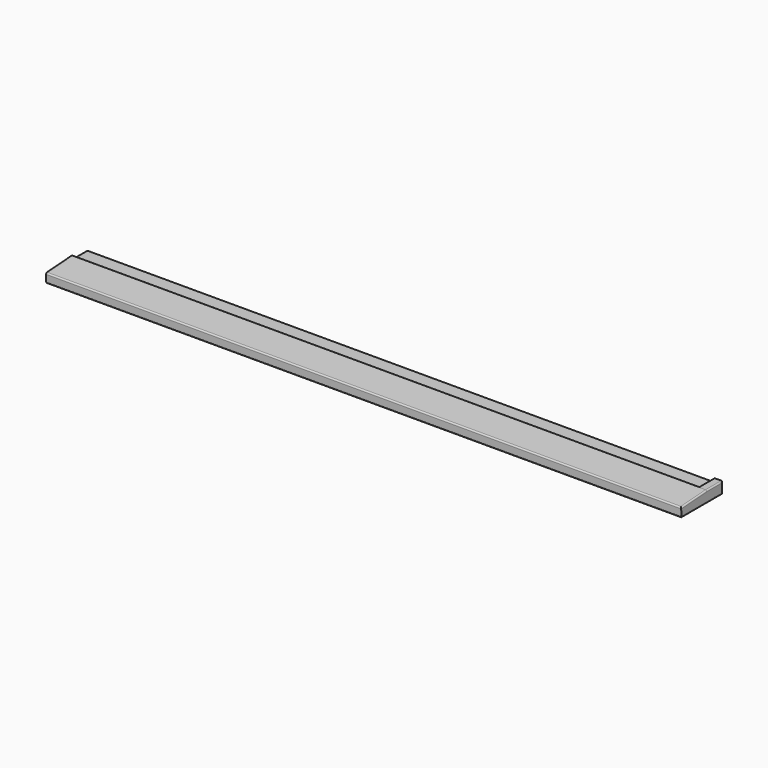
from build123d import *

# Parameters (mm, degrees)
F1_DEPTH    = 2390
F3_DEPTH    = 20
F5_DEPTH    = 10
F6_T1_DEPTH = 216.618628623
F6_T3_DEPTH = 142.4030805268
F6_T5_DEPTH = 100.344113211
F6_T7_DEPTH = 68.9770272469


# Not quite as in the source:
# - a fillet or chamfer that OpenCascade refuses, or shapes differently, is made with other operations: its cross-section is extruded or revolved along the edge and cut away or added


with BuildPart() as f1:
    # F0 (on Right) → F1 (new body)
    with BuildSketch(Plane.YZ):
        with BuildLine():
            Line((0, -19.8239199817), (0, 0))
            Line((0, 0), (190, 0))
            Line((190, 0), (190, 10))
            Line((190, 10), (120, 10))
            Line((120, 10), (120, 19.1649627105))
            ThreePointArc((120, 19.1649627105), (118.4117029432, 22.8201348033), (114.655886789, 24.1531072651))
            Line((114.655886789, 24.1531072651), (-2.4688205766, 16.0731170599))
            ThreePointArc((-2.4688205766, 16.0731170599), (-5.8715951564, 14.3956872139), (-7.1172645938, 10.8122596114))
            Line((-7.1172645938, 10.8122596114), (-6.3410848379, -15.7684031874))
            ThreePointArc((-6.3410848379, -15.7684031874), (-4.7310556973, -18.6708970152), (-1.618628623, -19.8239199817))
            Line((-1.618628623, -19.8239199817), (0, -19.8239199817))
        make_face()
    extrude(amount=-F1_DEPTH)

    # F2 (on face) → F3 (join)
    with BuildSketch(Plane.YZ):
        with BuildLine():
            ThreePointArc((-6.3410848379, -15.7684031874), (-4.7310556973, -18.6708970152), (-1.618628623, -19.8239199817))
            Line((-1.618628623, -19.8239199817), (0, -19.8239199817))
            Line((0, -19.8239199817), (0, 0))
            Line((0, 0), (190, 0))
            Line((190, 0), (190, 10))
            Line((190, 10), (120, 10))
            Line((120, 10), (120, 19.1649627105))
            ThreePointArc((120, 19.1649627105), (118.6551720927, 22.5766656537), (115.344113211, 24.1531072651))
            Line((115.344113211, 24.1531072651), (114.655886789, 24.1531072651))
            Line((114.655886789, 24.1531072651), (-2.4688205766, 16.0731170599))
            ThreePointArc((-2.4688205766, 16.0731170599), (-5.8715951564, 14.3956872139), (-7.1172645938, 10.8122596114))
            Line((-7.1172645938, 10.8122596114), (-6.3410848379, -15.7684031874))
        make_face()
        with BuildLine():
            Line((120, 10), (190, 10))
            Line((190, 10), (190, 24.1531072651))
            Line((190, 24.1531072651), (115.344113211, 24.1531072651))
            ThreePointArc((115.344113211, 24.1531072651), (118.6551720927, 22.5766656537), (120, 19.1649627105))
            Line((120, 19.1649627105), (120, 10))
        make_face()
    extrude(amount=F3_DEPTH)

    # F4 (on face) → F5 (join)
    with BuildSketch(Plane.YZ.offset(20)):
        with BuildLine():
            Line((190, -19.8239199817), (190, 0))
            Line((190, 0), (190, 24.1531072651))
            Line((190, 24.1531072651), (114.655886789, 24.1531072651))
            Line((114.655886789, 24.1531072651), (-2.4688205766, 16.0731170599))
            ThreePointArc((-2.4688205766, 16.0731170599), (-5.8715951564, 14.3956872139), (-7.1172645938, 10.8122596114))
            Line((-7.1172645938, 10.8122596114), (-6.3410848379, -15.7684031874))
            ThreePointArc((-6.3410848379, -15.7684031874), (-4.7310556973, -18.6708970152), (-1.618628623, -19.8239199817))
            Line((-1.618628623, -19.8239199817), (0, -19.8239199817))
            Line((0, -19.8239199817), (190, -19.8239199817))
        make_face()
    extrude(amount=F5_DEPTH)

    # F6: fillet of radius 5 on 4 edges, made by hand

    # F6_s2 → F6_t1 (cut)
    with BuildSketch(Plane.XZ.offset(-202.5)):
        with BuildLine():
            ThreePointArc((30, -14.8239199817), (28.5355339059, -18.3594538877), (25, -19.8239199817))
            Line((25, -19.8239199817), (30, -19.8239199817))
            Line((30, -19.8239199817), (30, -14.8239199817))
        make_face()
    extrude(amount=F6_T1_DEPTH, mode=Mode.SUBTRACT)

    # F6_s4 → F6_t3 (cut)
    with BuildSketch(Plane(origin=(0, 128.2415133818, 8.8468965716), x_dir=(1, 0, 0), z_dir=(0, -0.9976289109, -0.0688226422))):
        with BuildLine():
            ThreePointArc((25, 16.2049170229), (28.5355339059, 14.7404509288), (30, 11.2049170229))
            Line((30, 11.2049170229), (30, 16.2049170229))
            Line((30, 16.2049170229), (25, 16.2049170229))
        make_face()
    extrude(amount=F6_T3_DEPTH, mode=Mode.SUBTRACT)

    # F6_s6 → F6_t5 (cut)
    with BuildSketch(Plane.XZ.offset(-202.5)):
        with BuildLine():
            ThreePointArc((25, 24.1531072651), (28.5355339059, 22.6886411711), (30, 19.1531072651))
            Line((30, 19.1531072651), (30, 24.1531072651))
            Line((30, 24.1531072651), (25, 24.1531072651))
        make_face()
    extrude(amount=F6_T5_DEPTH, mode=Mode.SUBTRACT)

    # F6_s8 → F6_t7 (cut)
    with BuildSketch(Plane.XY.offset(-32.3239199817)):
        with BuildLine():
            ThreePointArc((25, 190), (28.5355339059, 188.5355339059), (30, 185))
            Line((30, 185), (30, 190))
            Line((30, 190), (25, 190))
        make_face()
    extrude(amount=F6_T7_DEPTH, mode=Mode.SUBTRACT)


solid = f1.part
